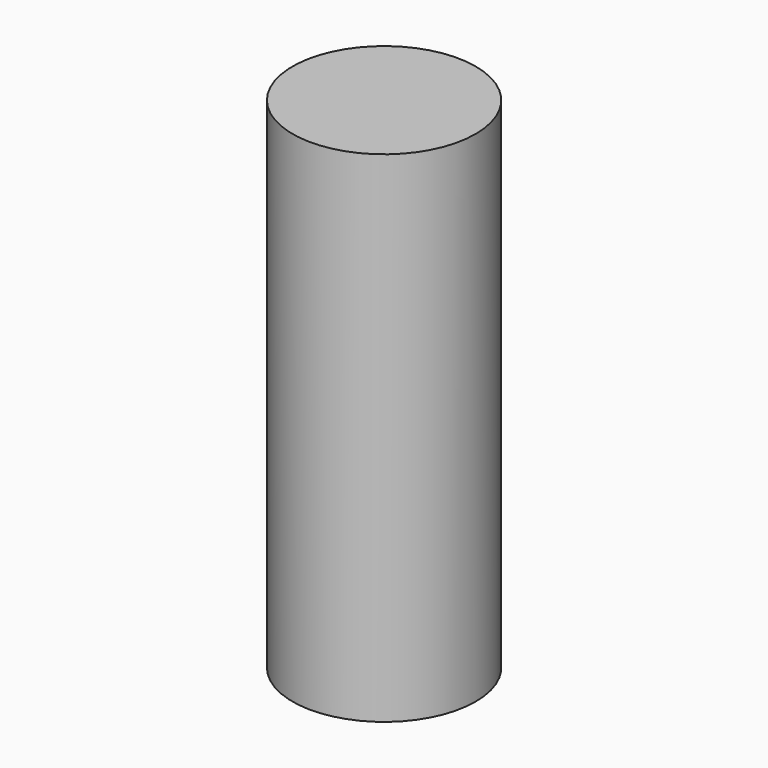
from build123d import *

# Parameters (mm, degrees)
F0_R     = 3700.0053
F1_DEPTH = 20200.00024


with BuildPart() as f1:
    # F0 (on Top) → F1 (new body)
    with BuildSketch(Plane.XY):
        Circle(F0_R)
    extrude(amount=F1_DEPTH)


solid = f1.part
